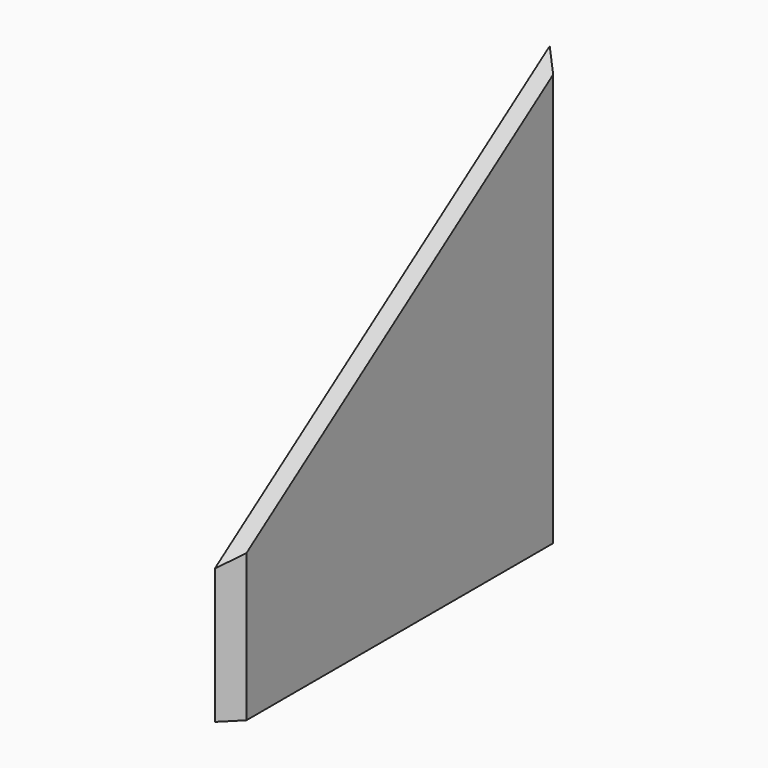
from build123d import *

# Parameters (mm, degrees)
F1_DEPTH    = 4.0000047
F2_T1_DEPTH = 112.2565983155
F3_T1_DEPTH = 247.2565983155


# Not quite as in the source:
# - a fillet or chamfer that OpenCascade refuses, or shapes differently, is made with other operations: its cross-section is extruded or revolved along the edge and cut away or added


with BuildPart() as f1:
    # F0 (on Right) → F1 (new body, symmetric)
    with BuildSketch(Plane.YZ):
        Polygon((-99.9751089393, -29.498891169), (-99.9751089393, -89.4988911689), (95.0248910607, -89.4988911689), (95.0248910607, 105.5011088311), align=None)
    extrude(amount=F1_DEPTH, both=True)

    # F2: chamfer of 10.16 on 1 edges, made by hand

    # F2_s2 → F2_t1 (cut)
    with BuildSketch(Plane.XY.offset(-115.6271903267)):
        Polygon((-6.1599953, -99.9751089393), (4.0000047, -89.8151089393), (4.0000047, -99.9751089393), align=None)
    extrude(amount=F2_T1_DEPTH, mode=Mode.SUBTRACT)

    # F3: chamfer of 10.16 on 1 edges, made by hand

    # F3_s2 → F3_t1 (cut)
    with BuildSketch(Plane.XY.offset(-115.6271903267)):
        Polygon((-6.1599953, 95.0248910607), (4.0000047, 84.8648910607), (4.0000047, 95.0248910607), align=None)
    extrude(amount=F3_T1_DEPTH, mode=Mode.SUBTRACT)


solid = f1.part
